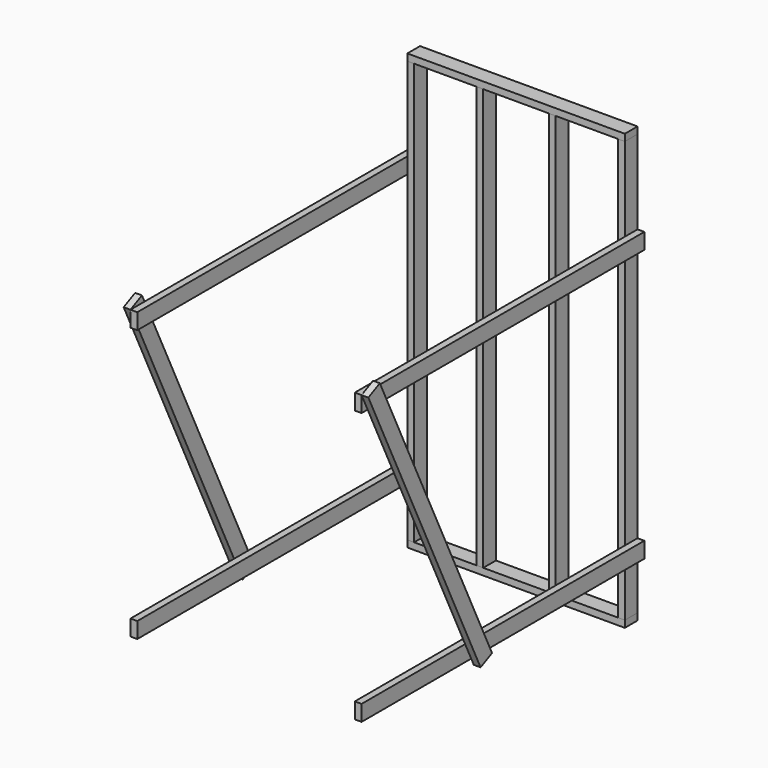
from build123d import *

# Parameters (mm, degrees)
F0_W      = 38.1
F0_H      = 2362.2
F1_DEPTH  = 88.9
F5_W      = 1219.2
F5_H      = 38.1
F6_DEPTH  = 88.9
F8_W      = 1828.8
F8_H      = 88.9
F9_DEPTH  = 38.1
F12_DEPTH = 38.1
F14_W     = 1981.2
F14_H     = 88.9
F15_DEPTH = 38.1
F20_DEPTH = 38.1


# Not quite as in the source:
# - a feature of the source that left no trace in its solid (it failed there, or was rolled back) is left out
# - a pattern or mirror of a feature is missing from the dataset's text; its kind, count and spacing are read off the source's solid


with BuildPart() as f1:
    # F0 (on Front) → F1 (new body)
    with BuildSketch(Plane.XZ):
        with Locations((19.05, 1181.1)):
            Rectangle(F0_W, F0_H)
    extrude(amount=F1_DEPTH)


with BuildPart() as f2_1:
    # F2: copy of F1
    add(f1.part.moved(Location((387.35, 0, 0))))


with BuildPart() as f3_1:
    # F3: copy of F2_1
    add(f2_1.part.moved(Location((406.4, 0, 0))))


with BuildPart() as f4_1:
    # F4: copy of F3_1
    add(f3_1.part.moved(Location((387.35, 0, 0))))


with BuildPart() as f6:
    # F5 (on Front) → F6 (new body)
    with BuildSketch(Plane.XZ):
        with Locations((609.6, -19.05)):
            Rectangle(F5_W, F5_H)
    extrude(amount=F6_DEPTH)


with BuildPart() as f6_copies_1:
    # F6_copies: instance of F6
    add(f6.part.mirror(Plane.XY.offset(1181.1)))


with BuildPart() as f9:
    # F8 (on face) → F9 (new body)
    with BuildSketch(Plane(origin=(0, 0, 0), x_dir=(0, -1, 0), z_dir=(-1, 0, 0))):
        with Locations((44.45, 6.35)):
            Rectangle(F8_W, F8_H)
    extrude(amount=F9_DEPTH)


with BuildPart() as f10_1:
    # F10: copy of F9
    add(f9.part.moved(Location((1257.3, 0, 0))))


with BuildPart() as f12:
    # F11 (on face) → F12 (new body)
    with BuildSketch(Plane(origin=(1219.2, 0, 0), x_dir=(0, -1, 0), z_dir=(-1, 0, 0))):
        Polygon((0, 1480.6079416481), (-825.5, 50.8), (-722.8471221381, 50.8), (0, 1302.8079416481), align=None)
        Polygon((88.9, 1634.587258441), (0, 1480.6079416481), (0, 1302.8079416481), (88.9, 1456.787258441), align=None)
    extrude(amount=-F12_DEPTH)


with BuildPart() as f13_1:
    # F13: copy of F12
    add(f12.part.moved(Location((-1257.3, 0, 0))))


with BuildPart() as f15:
    # F14 (on Right) → F15 (new body)
    with BuildSketch(Plane.YZ):
        with Locations((-990.6, 1847.85)):
            Rectangle(F14_W, F14_H)
    extrude(amount=-F15_DEPTH)


with BuildPart() as f16_1:
    # F16: copy of F15
    add(f15.part.moved(Location((1257.3, 0, 0))))


with BuildPart() as f17_1:
    # F17: copy of F15
    add(f15.part.moved(Location((0, 0, -1524))))


with BuildPart() as f18_1:
    # F18: copy of F17_1
    add(f17_1.part.moved(Location((1257.3, 0, 0))))


with BuildPart() as f20:
    # F19 (on face) → F20 (new body)
    with BuildSketch(Plane.YZ.offset(1257.3)):
        Polygon((-1114.616916851, 279.4), (-1900.9370329048, 1930.5238945304), (-1981.2, 1892.3), (-1194.8798839462, 241.1761054696), align=None)
    extrude(amount=F20_DEPTH)


with BuildPart() as f21_1:
    # F21: copy of F20
    add(f20.part.moved(Location((-1333.5, 0, 0))))


solid = Compound([f1.part, f2_1.part, f3_1.part, f4_1.part, f6.part, f6_copies_1.part, f15.part, f16_1.part, f17_1.part, f18_1.part, f20.part, f21_1.part])
